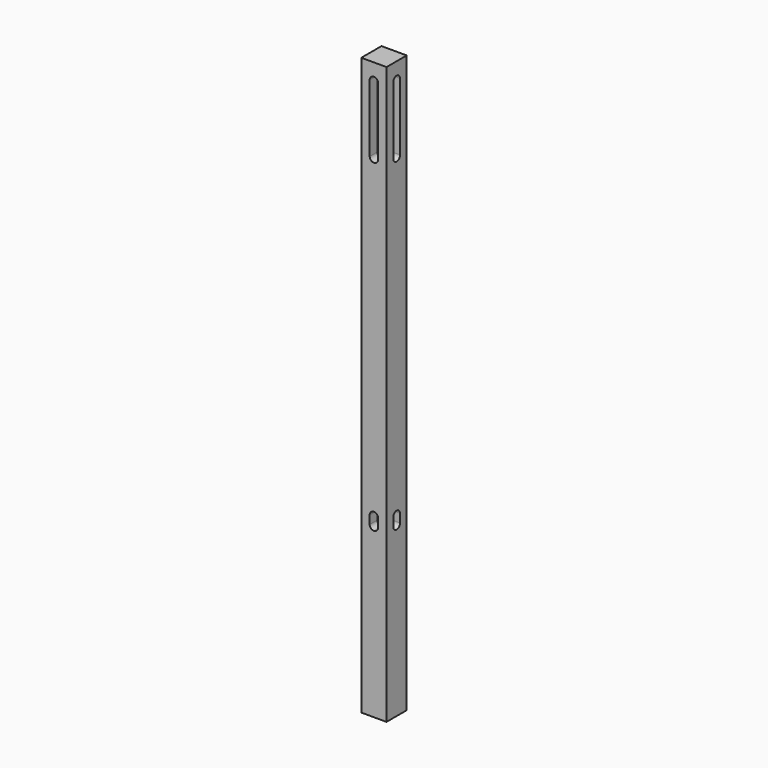
from build123d import *

# Parameters (mm, degrees)
F0_W         = 38.1
F0_H         = 38.1
F1_DEPTH     = 869.95
F2_W         = 12.7
F2_H         = 114.3
F2_H_2       = 25.4
F3_DEPTH     = 14.2875
F4_W         = 12.7
F4_H         = 114.3
F4_H_2       = 25.4
F5_DEPTH     = 14.2875
F6_T1_DEPTH  = 30.1625
F6_T3_DEPTH  = 12.7
F6_T5_DEPTH  = 30.1625
F6_T7_DEPTH  = 12.7
F6_T13_DEPTH = 28.575
F6_T17_DEPTH = 28.575
F6_T24_DEPTH = 28.575
F6_T28_DEPTH = 28.575
F6_T35_DEPTH = 28.575
F6_T39_DEPTH = 28.575
F6_T46_DEPTH = 28.575
F6_T50_DEPTH = 28.575


# Not quite as in the source:
# - a fillet or chamfer that OpenCascade refuses, or shapes differently, is made with other operations: its cross-section is extruded or revolved along the edge and cut away or added


with BuildPart() as f1:
    # F0 (on Top) → F1 (new body)
    with BuildSketch(Plane.XY):
        Rectangle(F0_W, F0_H)
    extrude(amount=-F1_DEPTH)

    # F2 (on face) → F3 (cut)
    with BuildSketch(Plane.XZ.offset(19.05)):
        with Locations((0, -76.2)):
            Rectangle(F2_W, F2_H)
        with Locations((0, -609.6)):
            Rectangle(F2_W, F2_H_2)
    extrude(amount=-F3_DEPTH, mode=Mode.SUBTRACT)

    # F4 (on face) → F5 (cut)
    with BuildSketch(Plane.YZ.offset(19.05)):
        with Locations((0, -76.2)):
            Rectangle(F4_W, F4_H)
        with Locations((0, -609.6)):
            Rectangle(F4_W, F4_H_2)
    extrude(amount=-F5_DEPTH, mode=Mode.SUBTRACT)

    # F6: fillet of radius 6.35 on 16 edges, made by hand

    # F6_s2 → F6_t1 (join)
    with BuildSketch(Plane.XZ.offset(-11.1125)):
        with BuildLine():
            ThreePointArc((-6.35, -25.4), (-4.4901280605, -20.9098719395), (0, -19.05))
            Line((0, -19.05), (-6.35, -19.05))
            Line((-6.35, -19.05), (-6.35, -25.4))
        make_face()
        with BuildLine():
            ThreePointArc((-6.35, -127), (-4.4901280605, -131.4901280605), (0, -133.35))
            Line((0, -133.35), (-6.35, -133.35))
            Line((-6.35, -133.35), (-6.35, -127))
        make_face()
        with BuildLine():
            ThreePointArc((-6.35, -603.25), (-4.4901280605, -598.7598719395), (0, -596.9))
            Line((0, -596.9), (-6.35, -596.9))
            Line((-6.35, -596.9), (-6.35, -603.25))
        make_face()
        with BuildLine():
            ThreePointArc((-6.35, -615.95), (-4.4901280605, -620.4401280605), (0, -622.3))
            Line((0, -622.3), (-6.35, -622.3))
            Line((-6.35, -622.3), (-6.35, -615.95))
        make_face()
    extrude(amount=F6_T1_DEPTH)

    # F6_s4 → F6_t3 (join)
    with BuildSketch(Plane.XZ.offset(6.35)):
        with BuildLine():
            ThreePointArc((6.35, -25.4), (4.4901280605, -20.9098719395), (0, -19.05))
            Line((0, -19.05), (6.35, -19.05))
            Line((6.35, -19.05), (6.35, -25.4))
        make_face()
        with BuildLine():
            ThreePointArc((0, -133.35), (4.4901280605, -131.4901280605), (6.35, -127))
            Line((6.35, -127), (6.35, -133.35))
            Line((6.35, -133.35), (0, -133.35))
        make_face()
        with BuildLine():
            ThreePointArc((6.35, -603.25), (4.4901280605, -598.7598719395), (0, -596.9))
            Line((0, -596.9), (6.35, -596.9))
            Line((6.35, -596.9), (6.35, -603.25))
        make_face()
        with BuildLine():
            ThreePointArc((0, -622.3), (4.4901280605, -620.4401280605), (6.35, -615.95))
            Line((6.35, -615.95), (6.35, -622.3))
            Line((6.35, -622.3), (0, -622.3))
        make_face()
    extrude(amount=F6_T3_DEPTH)

    # F6_s6 → F6_t5 (join)
    with BuildSketch(Plane.YZ.offset(-11.1125)):
        with BuildLine():
            ThreePointArc((0, -133.35), (4.4901280605, -131.4901280605), (6.35, -127))
            Line((6.35, -127), (6.35, -133.35))
            Line((6.35, -133.35), (0, -133.35))
        make_face()
        with BuildLine():
            ThreePointArc((0, -19.05), (4.4901280605, -20.9098719395), (6.35, -25.4))
            Line((6.35, -25.4), (6.35, -19.05))
            Line((6.35, -19.05), (0, -19.05))
        make_face()
        with BuildLine():
            ThreePointArc((0, -596.9), (4.4901280605, -598.7598719395), (6.35, -603.25))
            Line((6.35, -603.25), (6.35, -596.9))
            Line((6.35, -596.9), (0, -596.9))
        make_face()
        with BuildLine():
            ThreePointArc((0, -622.3), (4.4901280605, -620.4401280605), (6.35, -615.95))
            Line((6.35, -615.95), (6.35, -622.3))
            Line((6.35, -622.3), (0, -622.3))
        make_face()
    extrude(amount=F6_T5_DEPTH)

    # F6_s8 → F6_t7 (join)
    with BuildSketch(Plane.YZ.offset(6.35)):
        with BuildLine():
            ThreePointArc((0, -133.35), (-4.4901280605, -131.4901280605), (-6.35, -127))
            Line((-6.35, -127), (-6.35, -133.35))
            Line((-6.35, -133.35), (0, -133.35))
        make_face()
        with BuildLine():
            ThreePointArc((0, -19.05), (-4.4901280605, -20.9098719395), (-6.35, -25.4))
            Line((-6.35, -25.4), (-6.35, -19.05))
            Line((-6.35, -19.05), (0, -19.05))
        make_face()
        with BuildLine():
            ThreePointArc((0, -596.9), (-4.4901280605, -598.7598719395), (-6.35, -603.25))
            Line((-6.35, -603.25), (-6.35, -596.9))
            Line((-6.35, -596.9), (0, -596.9))
        make_face()
        with BuildLine():
            ThreePointArc((0, -622.3), (-4.4901280605, -620.4401280605), (-6.35, -615.95))
            Line((-6.35, -615.95), (-6.35, -622.3))
            Line((-6.35, -622.3), (0, -622.3))
        make_face()
    extrude(amount=F6_T7_DEPTH)


with BuildPart() as f6_tool11:
    # F6_s12 → F6_t13 (new body)
    with BuildSketch(Plane.XZ.offset(19.05)):
        with BuildLine():
            ThreePointArc((6.35, -25.4), (4.4901280605, -20.9098719395), (0, -19.05))
            Line((0, -19.05), (6.35, -19.05))
            Line((6.35, -19.05), (6.35, -25.4))
        make_face()
    extrude(amount=-F6_T13_DEPTH)

    split(bisect_by=Plane.XZ.offset(6.35), keep=Keep.BOTTOM)


with BuildPart() as f6_tool15:
    # F6_s16 → F6_t17 (new body)
    with BuildSketch(Plane.YZ.offset(19.05)):
        with BuildLine():
            ThreePointArc((0, -19.05), (-4.4901280605, -20.9098719395), (-6.35, -25.4))
            Line((-6.35, -25.4), (-6.35, -19.05))
            Line((-6.35, -19.05), (0, -19.05))
        make_face()
    extrude(amount=-F6_T17_DEPTH)

    split(bisect_by=Plane.YZ.offset(6.35), keep=Keep.BOTTOM)


with BuildPart() as f6_tool11_1:
    add(f6_tool11.part)

    # F6_t19: intersect F6_tool15
    add(f6_tool15.part, mode=Mode.INTERSECT)


with BuildPart() as f1_1:
    add(f1.part)

    # F6_t9: union F6_tool11
    add(f6_tool11_1.part)


with BuildPart() as f6_tool22:
    # F6_s23 → F6_t24 (new body)
    with BuildSketch(Plane.YZ.offset(19.05)):
        with BuildLine():
            ThreePointArc((0, -133.35), (-4.4901280605, -131.4901280605), (-6.35, -127))
            Line((-6.35, -127), (-6.35, -133.35))
            Line((-6.35, -133.35), (0, -133.35))
        make_face()
    extrude(amount=-F6_T24_DEPTH)

    split(bisect_by=Plane.YZ.offset(6.35), keep=Keep.BOTTOM)


with BuildPart() as f6_tool26:
    # F6_s27 → F6_t28 (new body)
    with BuildSketch(Plane.XZ.offset(19.05)):
        with BuildLine():
            ThreePointArc((0, -133.35), (4.4901280605, -131.4901280605), (6.35, -127))
            Line((6.35, -127), (6.35, -133.35))
            Line((6.35, -133.35), (0, -133.35))
        make_face()
    extrude(amount=-F6_T28_DEPTH)

    split(bisect_by=Plane.XZ.offset(6.35), keep=Keep.BOTTOM)


with BuildPart() as f6_tool22_1:
    add(f6_tool22.part)

    # F6_t30: intersect F6_tool26
    add(f6_tool26.part, mode=Mode.INTERSECT)


with BuildPart() as f1_2:
    add(f1_1.part)

    # F6_t20: union F6_tool22
    add(f6_tool22_1.part)


with BuildPart() as f6_tool33:
    # F6_s34 → F6_t35 (new body)
    with BuildSketch(Plane.XZ.offset(19.05)):
        with BuildLine():
            ThreePointArc((6.35, -603.25), (4.4901280605, -598.7598719395), (0, -596.9))
            Line((0, -596.9), (6.35, -596.9))
            Line((6.35, -596.9), (6.35, -603.25))
        make_face()
    extrude(amount=-F6_T35_DEPTH)

    split(bisect_by=Plane.XZ.offset(6.35), keep=Keep.BOTTOM)


with BuildPart() as f6_tool37:
    # F6_s38 → F6_t39 (new body)
    with BuildSketch(Plane.YZ.offset(19.05)):
        with BuildLine():
            ThreePointArc((0, -596.9), (-4.4901280605, -598.7598719395), (-6.35, -603.25))
            Line((-6.35, -603.25), (-6.35, -596.9))
            Line((-6.35, -596.9), (0, -596.9))
        make_face()
    extrude(amount=-F6_T39_DEPTH)

    split(bisect_by=Plane.YZ.offset(6.35), keep=Keep.BOTTOM)


with BuildPart() as f6_tool33_1:
    add(f6_tool33.part)

    # F6_t41: intersect F6_tool37
    add(f6_tool37.part, mode=Mode.INTERSECT)


with BuildPart() as f1_3:
    add(f1_2.part)

    # F6_t31: union F6_tool33
    add(f6_tool33_1.part)


with BuildPart() as f6_tool44:
    # F6_s45 → F6_t46 (new body)
    with BuildSketch(Plane.YZ.offset(19.05)):
        with BuildLine():
            ThreePointArc((0, -622.3), (-4.4901280605, -620.4401280605), (-6.35, -615.95))
            Line((-6.35, -615.95), (-6.35, -622.3))
            Line((-6.35, -622.3), (0, -622.3))
        make_face()
    extrude(amount=-F6_T46_DEPTH)

    split(bisect_by=Plane.YZ.offset(6.35), keep=Keep.BOTTOM)


with BuildPart() as f6_tool48:
    # F6_s49 → F6_t50 (new body)
    with BuildSketch(Plane.XZ.offset(19.05)):
        with BuildLine():
            ThreePointArc((0, -622.3), (4.4901280605, -620.4401280605), (6.35, -615.95))
            Line((6.35, -615.95), (6.35, -622.3))
            Line((6.35, -622.3), (0, -622.3))
        make_face()
    extrude(amount=-F6_T50_DEPTH)

    split(bisect_by=Plane.XZ.offset(6.35), keep=Keep.BOTTOM)


with BuildPart() as f6_tool44_1:
    add(f6_tool44.part)

    # F6_t52: intersect F6_tool48
    add(f6_tool48.part, mode=Mode.INTERSECT)


with BuildPart() as f1_4:
    add(f1_3.part)

    # F6_t42: union F6_tool44
    add(f6_tool44_1.part)


solid = f1_4.part
